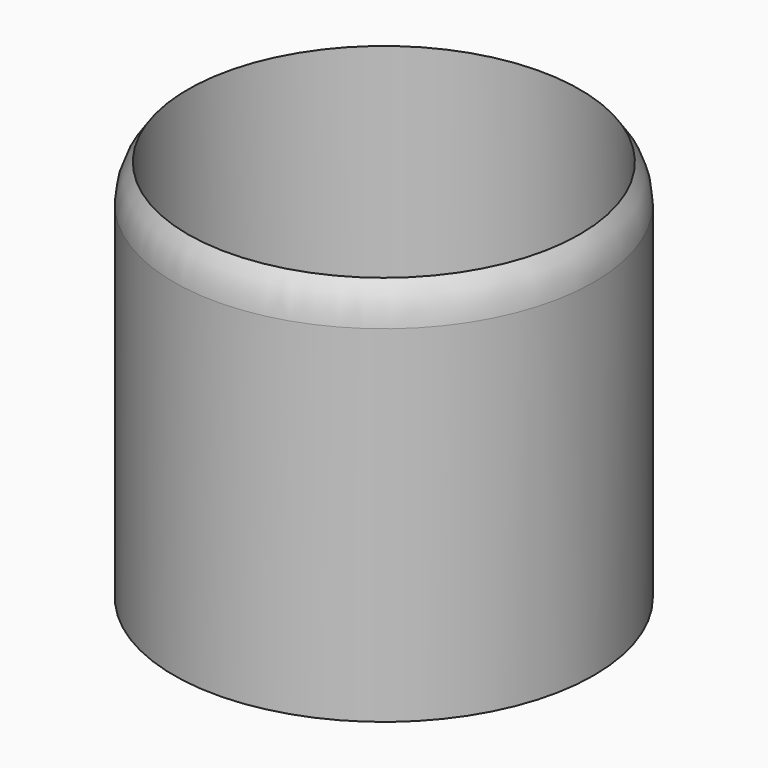
from build123d import *

# Parameters (mm, degrees)
F0_R     = 38.1
F1_DEPTH = 34.798
F2_T     = -2.54


# Not quite as in the source:
# - a fillet or chamfer that OpenCascade refuses, or shapes differently, is made with other operations: its cross-section is extruded or revolved along the edge and cut away or added
# - the program builds the solid bodies; features that only make, move or delete a surface that nothing else refers to are left out


with BuildPart() as f1:
    # F0 (on Top) → F1 (new body, symmetric)
    with BuildSketch(Plane.XY):
        Circle(F0_R)
    extrude(amount=F1_DEPTH, both=True)

    # F2
    f2_openings = [f1.faces().sort_by_distance(p)[0] for p in [
        (0, 0, 34.798),
    ]]
    offset(amount=F2_T, openings=f2_openings)

    # F3: fillet of radius 10.4245741623 on 1 edges, made by hand

    # F3_s1 → F3_t2 (revolve, cut)
    with BuildSketch(Plane.XZ):
        with BuildLine():
            ThreePointArc((38.1, 27.9785251856), (37.4443836777, 31.617097596), (35.56, 34.798))
            Line((35.56, 34.798), (38.1, 34.798))
            Line((38.1, 34.798), (38.1, 27.9785251856))
        make_face()
    revolve(axis=Axis((0, 0, 34.798), (0, 0, 1)), mode=Mode.SUBTRACT)


solid = f1.part
